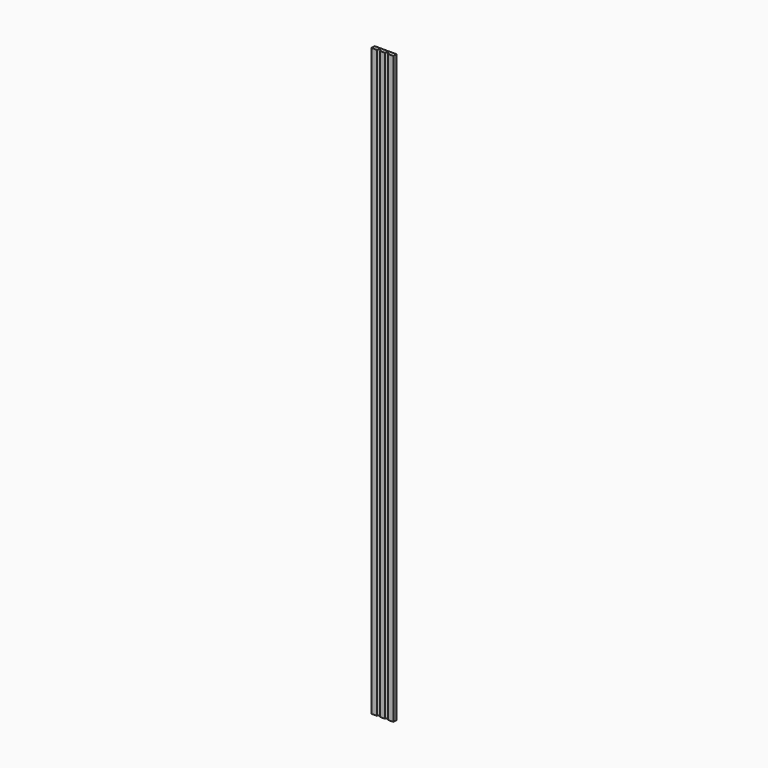
from build123d import *

# Parameters (mm, degrees)
F1_W     = 88.9
F1_H     = 2374.9
F2_DEPTH = 15.875
F4_DEPTH = 2374.9


# Not quite as in the source:
# - a variable given as a bare number and used for a length is read in inches; the dataset says mm whatever the document's units were
# - a length typed as a fraction of an inch, garbled in the dataset ("3 / 203.2 mm" for 3/8 in), is restored


with BuildPart() as f2:
    # F1 (on Front) → F2 (new body)
    with BuildSketch(Plane.XZ):
        with Locations((44.45, 1187.45)):
            Rectangle(F1_W, F1_H)
    extrude(amount=F2_DEPTH)

    # F3 (on Top) → F4 (cut)
    with BuildSketch(Plane.XY):
        with BuildLine():
            Line((22.225, -15.875), (34.925, -15.875))
            ThreePointArc((34.925, -15.875), (28.575, -9.525), (22.225, -15.875))
        make_face()
        with BuildLine():
            Line((53.975, -15.875), (66.675, -15.875))
            ThreePointArc((66.675, -15.875), (60.325, -9.525), (53.975, -15.875))
        make_face()
    extrude(amount=F4_DEPTH, mode=Mode.SUBTRACT)


solid = f2.part
